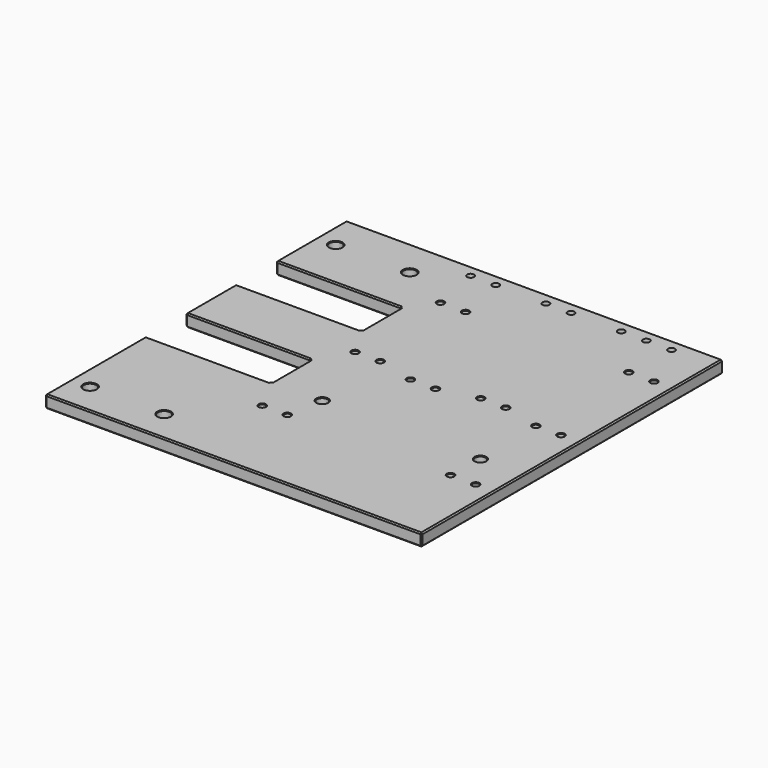
from build123d import *

# Parameters (mm, degrees)
F0_W      = 300
F0_H      = 10
F1_DEPTH  = 300
F3_DEPTH  = 10.001
F4_SIZE   = 1
F5_R      = 2.5
F6_DEPTH  = 25
F7_SIZE   = 0.5
F8_R      = 5
F9_DEPTH  = 10.001
F10_SIZE  = 0.5
F11_R     = 4.25
F12_DEPTH = 10.001
F13_SIZE  = 0.5
F14_R     = 2.75
F15_DEPTH = 10.001


# Not quite as in the source:
# - a feature names something its author has since deleted; it is built from what else it names


with BuildPart() as f1:
    # F0 (on Right) → F1 (new body)
    with BuildSketch(Plane.YZ):
        with Locations((-150, 5)):
            Rectangle(F0_W, F0_H)
    extrude(amount=-F1_DEPTH)

    # F2 (on face) → F3 (cut, through all)
    with BuildSketch(Plane.XY.offset(10)):
        Polygon((-200, -70), (-300, -70), (-300, -110), (-200, -110), (-200, -90), align=None)
        Polygon((-200, -160), (-300, -160), (-300, -200), (-200, -200), (-200, -180), align=None)
    extrude(amount=-F3_DEPTH, mode=Mode.SUBTRACT)

    # F4
    f4_edges = [f1.edges().sort_by_distance(p)[0] for p in [
        (0, -150, 10),
        (-150, -300, 10),
        (-300, -250, 10),
        (-250, -200, 10),
        (-200, -180, 10),
        (-250, -160, 10),
        (-300, -135, 10),
        (-250, -110, 10),
        (-200, -90, 10),
        (-250, -70, 10),
        (-300, -35, 10),
        (-150, 0, 10),
        (0, -150, 0),
        (-150, 0, 0),
        (-300, -35, 0),
        (-250, -70, 0),
        (-200, -90, 0),
        (-250, -110, 0),
        (-300, -135, 0),
        (-250, -160, 0),
        (-200, -180, 0),
        (-250, -200, 0),
        (-300, -250, 0),
        (-150, -300, 0),
        (0, -300, 5),
        (0, 0, 5),
        (-300, -70, 5),
        (-200, -70, 5),
        (-200, -110, 5),
        (-300, -110, 5),
        (-300, -160, 5),
        (-200, -160, 5),
        (-200, -200, 5),
        (-300, -200, 5),
        (-300, -300, 5),
    ]]
    chamfer(f4_edges, length=F4_SIZE)

    # F5 (on face) → F6 (cut)
    with BuildSketch(Plane.XY.offset(10)):
        with Locations((-15, -50)):
            Circle(F5_R)
        with Locations((-35, -50)):
            Circle(F5_R)
        with Locations((-165, -50)):
            Circle(F5_R)
        with Locations((-185, -50)):
            Circle(F5_R)
        with Locations((-65, -135)):
            Circle(F5_R)
        with Locations((-85, -135)):
            Circle(F5_R)
        with Locations((-165, -135)):
            Circle(F5_R)
        with Locations((-185, -135)):
            Circle(F5_R)
        with Locations((-15, -227.5)):
            Circle(F5_R)
        with Locations((-35, -227.5)):
            Circle(F5_R)
        with Locations((-165, -227.5)):
            Circle(F5_R)
        with Locations((-185, -227.5)):
            Circle(F5_R)
        with Locations((-15, -142.5)):
            Circle(F5_R)
        with Locations((-35, -142.5)):
            Circle(F5_R)
        with Locations((-115, -142.5)):
            Circle(F5_R)
        with Locations((-135, -142.5)):
            Circle(F5_R)
    extrude(amount=-F6_DEPTH, mode=Mode.SUBTRACT)

    # F7
    f7_edges = [f1.edges().sort_by_distance(p)[0] for p in [
        (-17.5, -50, 10),
        (-12.5, -50, 5),
        (-17.5, -50, 0),
        (-37.5, -50, 10),
        (-32.5, -50, 5),
        (-37.5, -50, 0),
        (-167.5, -50, 10),
        (-162.5, -50, 5),
        (-167.5, -50, 0),
        (-187.5, -50, 10),
        (-182.5, -50, 5),
        (-187.5, -50, 0),
        (-67.5, -135, 10),
        (-62.5, -135, 5),
        (-67.5, -135, 0),
        (-87.5, -135, 10),
        (-82.5, -135, 5),
        (-87.5, -135, 0),
        (-187.5, -135, 10),
        (-182.5, -135, 5),
        (-187.5, -135, 0),
        (-167.5, -135, 10),
        (-162.5, -135, 5),
        (-167.5, -135, 0),
        (-17.5, -142.5, 10),
        (-12.5, -142.5, 5),
        (-17.5, -142.5, 0),
        (-37.5, -142.5, 10),
        (-32.5, -142.5, 5),
        (-37.5, -142.5, 0),
        (-117.5, -142.5, 10),
        (-112.5, -142.5, 5),
        (-117.5, -142.5, 0),
        (-137.5, -142.5, 10),
        (-132.5, -142.5, 5),
        (-137.5, -142.5, 0),
        (-17.5, -227.5, 10),
        (-12.5, -227.5, 5),
        (-17.5, -227.5, 0),
        (-37.5, -227.5, 10),
        (-32.5, -227.5, 5),
        (-37.5, -227.5, 0),
        (-167.5, -227.5, 10),
        (-162.5, -227.5, 5),
        (-167.5, -227.5, 0),
        (-187.5, -227.5, 10),
        (-182.5, -227.5, 5),
        (-187.5, -227.5, 0),
    ]]
    chamfer(f7_edges, length=F7_SIZE)

    # F8 (on face) → F9 (cut, through all)
    with BuildSketch(Plane.XY.offset(10)):
        with Locations((-284.5, -274.6)):
            Circle(F8_R)
        with Locations((-225.5, -274.6)):
            Circle(F8_R)
        with Locations((-284.5, -30)):
            Circle(F8_R)
        with Locations((-225.5, -30)):
            Circle(F8_R)
    extrude(amount=-F9_DEPTH, mode=Mode.SUBTRACT)

    # F10
    f10_edges = [f1.edges().sort_by_distance(p)[0] for p in [
        (-289.5, -30, 10),
        (-279.5, -30, 5),
        (-289.5, -30, 0),
        (-230.5, -30, 10),
        (-220.5, -30, 5),
        (-230.5, -30, 0),
        (-289.5, -274.6, 10),
        (-279.5, -274.6, 5),
        (-289.5, -274.6, 0),
        (-230.5, -274.6, 10),
        (-220.5, -274.6, 5),
        (-230.5, -274.6, 0),
    ]]
    chamfer(f10_edges, length=F10_SIZE)

    # F11 (on face) → F12 (cut, through all)
    with BuildSketch(Plane.XY.offset(10)):
        with Locations((-34, -199)):
            Circle(F11_R)
        with Locations((-160, -199)):
            Circle(F11_R)
    extrude(amount=-F12_DEPTH, mode=Mode.SUBTRACT)

    # F13
    f13_edges = [f1.edges().sort_by_distance(p)[0] for p in [
        (-164.25, -199, 10),
        (-155.75, -199, 5),
        (-164.25, -199, 0),
        (-38.25, -199, 10),
        (-29.75, -199, 5),
        (-38.25, -199, 0),
    ]]
    chamfer(f13_edges, length=F13_SIZE)

    # F14 (on face) → F15 (cut, through all)
    with BuildSketch(Plane.XY.offset(10)):
        with Locations((-193, -10)):
            Circle(F14_R)
        with Locations((-173, -10)):
            Circle(F14_R)
        with Locations((-133, -10)):
            Circle(F14_R)
        with Locations((-113, -10)):
            Circle(F14_R)
        with Locations((-73, -10)):
            Circle(F14_R)
        with Locations((-53, -10)):
            Circle(F14_R)
        with Locations((-33, -10)):
            Circle(F14_R)
    extrude(amount=-F15_DEPTH, mode=Mode.SUBTRACT)


solid = f1.part
